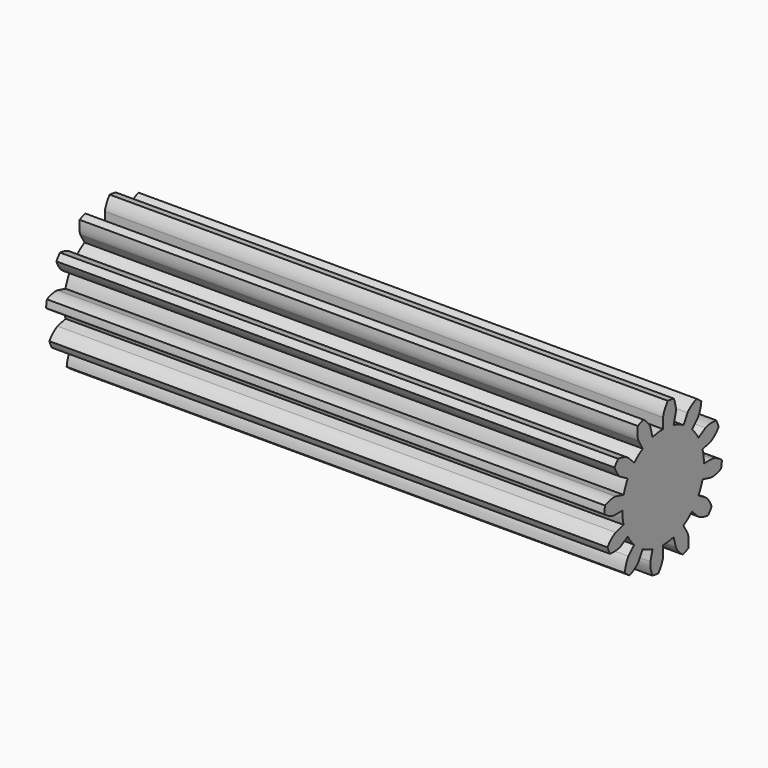
from build123d import *

# Parameters (mm, degrees)
F3_DEPTH        = 40
F3_COPIES_COUNT = 12


# Not quite as in the source:
# - a feature of the source that left no trace in its solid (it failed there, or was rolled back) is left out
# - a pattern or mirror of a feature is missing from the dataset's text; its kind, count and spacing are read off the source's solid
# - a feature names something its author has since deleted; it is built from what else it names


with BuildPart() as f3:
    # F2 (on Right) → F3 (new body)
    with BuildSketch(Plane.YZ):
        with BuildLine():
            ThreePointArc((-3.6579282742, 0), (0, -3.6579282742), (3.6579282742, 0))
            ThreePointArc((3.6579282742, 0), (0.477455449, 3.6266341908), (-3.5332873908, 0.946741503))
            ThreePointArc((-3.5332873908, 0.946741503), (-3.6266341908, 0.477455449), (-3.6579282742, 0))
        make_face()
        with BuildLine():
            ThreePointArc((-3.6579282742, 0), (-3.6266341908, 0.477455449), (-3.5332873908, 0.946741503))
            Line((-3.5332873908, 0.946741503), (-4.2379647122, 1.1355592222))
            add(Edge.make_bspline(
                [(-4.2379647122, 1.1355592222), (-4.2437467288, 1.1371085089), (-4.2403131347, 1.1360287117), (-4.2622061027, 1.1406237524), (-4.2869304563, 1.1437141255), (-4.3260113323, 1.1472646892), (-4.3750726811, 1.1490077252), (-4.435495523, 1.1482332327), (-4.5066411711, 1.1437228755), (-4.588420692, 1.1344250199), (-4.6804022829, 1.1192894198), (-4.7824332878, 1.0971614297), (-4.8930433203, 1.0674823467), (-5.0155948084, 1.027429312), (-5.1089164916, 0.9926582339), (-5.1806954565, 0.961948838), (-5.2004561199, 0.9533315859)],
                knots=[0, 0, 0, 0, 0.0202164122, 0.055231725, 0.1004362437, 0.1539229332, 0.2145711301, 0.2816202297, 0.3545102827, 0.4328067574, 0.5161597183, 0.6042794907, 0.6969211254, 0.7938739525, 0.8949542617, 0.9361504501, 0.9361504501, 0.9361504501, 0.9361504501], degree=3))
            ThreePointArc((-5.2004561199, 0.9533315859), (-5.241882993, 0.6901069881), (-5.2699952454, 0.4251294873))
            add(Edge.make_bspline(
                [(-4.3874639199, 0), (-4.393449904, 0), (-4.3898538347, 0.0001543244), (-4.4121901019, 0.001382173), (-4.436871841, 0.0047962354), (-4.475540022, 0.0114815293), (-4.5233807768, 0.0224958972), (-4.5815443069, 0.0388825818), (-4.6490983595, 0.061653101), (-4.7256848487, 0.0918002373), (-4.8106148613, 0.1302266919), (-4.9034420988, 0.1780082563), (-5.0026016739, 0.235304032), (-5.1106108331, 0.3057109518), (-5.1917532398, 0.3634506631), (-5.2531382193, 0.4116914248), (-5.2699952454, 0.4251294873)],
                knots=[0, 0, 0, 0, 0.0202164122, 0.055231725, 0.1004362437, 0.1539229332, 0.2145711301, 0.2816202297, 0.3545102827, 0.4328067574, 0.5161597183, 0.6042794907, 0.6969211254, 0.7938739525, 0.8949542617, 0.9361504501, 0.9361504501, 0.9361504501, 0.9361504501], degree=3))
            Line((-4.3874639199, 0), (-3.6579282742, 0))
        make_face()
    extrude(amount=F3_DEPTH)

    # F3_copies: F3 ×12 about axis
    f3_copies_axis = Axis((0, 0, 0), (1, 0, 0))


with BuildPart() as f3_1:
    add(f3.part)
    for i in range(1, F3_COPIES_COUNT):
        add(f3.part.rotate(f3_copies_axis, i * 360 / F3_COPIES_COUNT))


solid = f3_1.part
